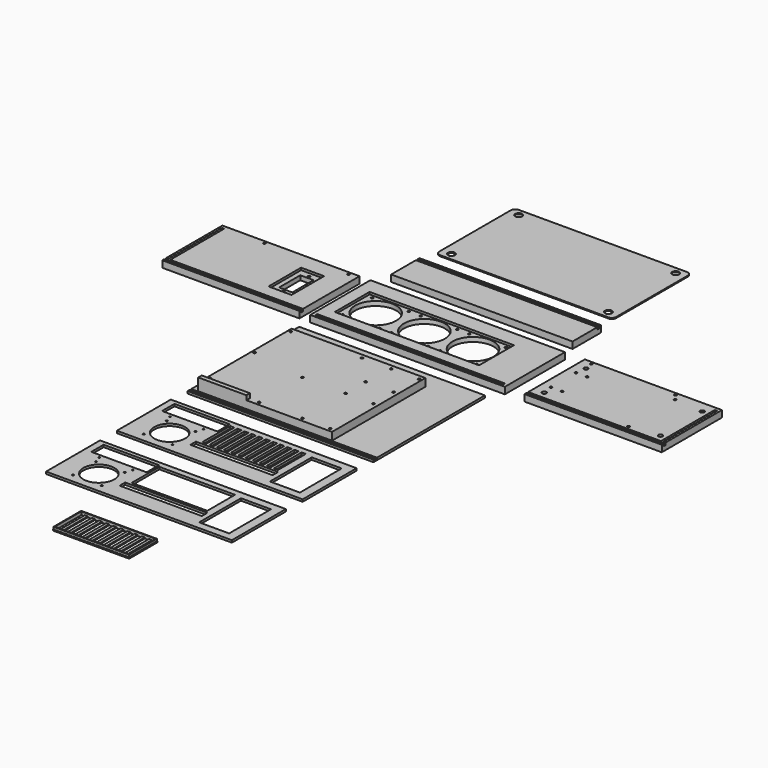
from build123d import *

# Parameters (mm, degrees)
F0_W      = 558.8
F0_H      = 215.9
F0_W_2    = 539.75
F0_H_2    = 6.5278
F0_W_3    = 414.33164
F0_H_3    = 125
F0_R      = 3.1877
F0_R_2    = 59
F1_DEPTH  = 12.7
F2_DEPTH  = 6.35
F3_R      = 6
F3_R_2    = 3.302
F3_W      = 393.7
F3_H      = 6.35
F3_W_2    = 6.3754
F3_H_2    = 2.8363937142
F3_H_3    = 193.4972
F4_DEPTH  = 12.7
F5_DEPTH  = 6.35
F6_R      = 3.302
F6_W      = 66.04
F6_H      = 116.84
F6_W_2    = 38.1
F6_H_2    = 76.2
F6_W_3    = 393.7
F6_H_3    = 6.35
F6_W_4    = 6.3754
F6_H_4    = 193.4972
F6_H_5    = 3.974708319
F7_DEPTH  = 12.7
F8_DEPTH  = 6.35
F9_DEPTH  = 6.35
F10_R     = 3.302
F10_W     = 138.0889187211
F10_H     = 12.6182494217
F11_DEPTH = 25.4
F12_DEPTH = 38.1
F13_W     = 533.4
F13_H     = 387.1722
F13_R     = 3.302
F13_H_2   = 6.5278
F13_H_3   = 6.35
F14_DEPTH = 3.2
F15_DEPTH = 3.2
F16_W     = 533.4
F16_H     = 193.6500064
F16_R     = 2.5
F16_R_2   = 44.5
F16_W_2   = 236.050014
F16_H_2   = 20
F16_R_3   = 2.0970704069
F16_R_4   = 2.1817303996
F16_W_3   = 12.0000014
F16_H_3   = 99.38
F16_W_4   = 158.75
F16_H_4   = 44.45
F16_W_5   = 12
F16_W_6   = 86
F16_H_5   = 150
F17_DEPTH = 6.3754
F18_W     = 520.7
F18_H     = 88.7222
F18_H_2   = 6.5278
F18_H_3   = 6.35
F19_DEPTH = 12.7
F20_DEPTH = 6.35
F21_R     = 10
F22_DEPTH = 3
F23_W     = 533.4
F23_H     = 193.6500064
F23_R     = 2.5
F23_R_2   = 44.5
F23_W_2   = 236.050014
F23_H_2   = 20
F23_R_3   = 2.0970704069
F23_R_4   = 2.1817303996
F23_W_3   = 158.75
F23_H_3   = 44.45
F23_W_4   = 217.000014
F23_H_4   = 99.38
F23_W_5   = 86
F23_H_5   = 150
F24_DEPTH = 6.3754
F25_W     = 219.000014
F25_H     = 101.3799892
F25_W_2   = 217.000014
F25_H_2   = 99.3799892
F25_W_3   = 8.5000084
F25_H_3   = 95.3799892
F25_W_4   = 8.499923
F26_DEPTH = 3
F27_DEPTH = 9.4


# Not quite as in the source:
# - a feature names something its author has since deleted; it is built from what else it names


with BuildPart() as f1:
    # F0 (on Top) → F1 (new body)
    with BuildSketch(Plane.XY):
        Rectangle(F0_W, F0_H)
        with Locations((0, -98.3361)):
            Rectangle(F0_W_2, F0_H_2, mode=Mode.SUBTRACT)
        with Locations((-38.1, 0)):
            Rectangle(F0_W_3, F0_H_3, mode=Mode.SUBTRACT)
        with Locations((-38.1, 0)):
            Rectangle(F0_W_3, F0_H_3)
        with Locations((-230.3, -52.5)):
            Circle(F0_R, mode=Mode.SUBTRACT)
        with Locations((-125.3, -52.5)):
            Circle(F0_R, mode=Mode.SUBTRACT)
        with Locations((-90.6, -52.5)):
            Circle(F0_R, mode=Mode.SUBTRACT)
        with Locations((14.4, -52.5)):
            Circle(F0_R, mode=Mode.SUBTRACT)
        with Locations((49.1, -52.5)):
            Circle(F0_R, mode=Mode.SUBTRACT)
        with Locations((154.1, -52.5)):
            Circle(F0_R, mode=Mode.SUBTRACT)
        with Locations((-177.8, 0)):
            Circle(F0_R_2, mode=Mode.SUBTRACT)
        with Locations((-230.3, 52.5)):
            Circle(F0_R, mode=Mode.SUBTRACT)
        with Locations((-38.1, 0)):
            Circle(F0_R_2, mode=Mode.SUBTRACT)
        with Locations((-125.3, 52.5)):
            Circle(F0_R, mode=Mode.SUBTRACT)
        with Locations((-90.6, 52.5)):
            Circle(F0_R, mode=Mode.SUBTRACT)
        with Locations((101.6, 0)):
            Circle(F0_R_2, mode=Mode.SUBTRACT)
        with Locations((14.4, 52.5)):
            Circle(F0_R, mode=Mode.SUBTRACT)
        with Locations((49.1, 52.5)):
            Circle(F0_R, mode=Mode.SUBTRACT)
        with Locations((154.1, 52.5)):
            Circle(F0_R, mode=Mode.SUBTRACT)
        with Locations((0, -98.3361)):
            Rectangle(F0_W_2, F0_H_2)
    extrude(amount=-F1_DEPTH)

    # F0 (on Top) → F2 (join)
    with BuildSketch(Plane.XY):
        Rectangle(F0_W, F0_H)
        with Locations((0, -98.3361)):
            Rectangle(F0_W_2, F0_H_2, mode=Mode.SUBTRACT)
        with Locations((-38.1, 0)):
            Rectangle(F0_W_3, F0_H_3, mode=Mode.SUBTRACT)
    extrude(amount=F2_DEPTH)


with BuildPart() as f4:
    # F3 (on Top) → F4 (new body)
    with BuildSketch(Plane.XY):
        Polygon((336.1011743546, 107.95), (336.1011743546, -95.0722), (717.0757743546, -95.0722), (717.0757743546, 98.425), (723.4511743546, 98.425), (723.4511743546, -95.0722), (729.8011743546, -95.0722), (729.8011743546, 107.95), align=None)
        with Locations((366.1011743546, -74.95)):
            Circle(F3_R, mode=Mode.SUBTRACT)
        with BuildLine():
            Line((389.9992377546, -45.0850025), (364.8031743546, -45.0850025))
            ThreePointArc((364.8031743546, -45.0850025), (359.1663077631, -47.4198690915), (361.5011743546, -41.7830025))
            Line((361.5011743546, -41.7830025), (361.5011743546, 41.7829975))
            ThreePointArc((361.5011743546, 41.7829975), (359.1663077631, 47.4198640915), (364.8031743546, 45.0849975))
            Line((364.8031743546, 45.0849975), (389.9992377546, 45.0849975))
            ThreePointArc((389.9992377546, 45.0849975), (393.3012377546, 48.3869975), (396.6032377546, 45.0849975))
            ThreePointArc((396.6032377546, 45.0849975), (395.636104346, 42.7501309085), (393.3012377546, 41.7829975))
            Line((393.3012377546, 41.7829975), (393.3012377546, -41.7830025))
            ThreePointArc((393.3012377546, -41.7830025), (395.636104346, -42.7501359085), (396.6032377546, -45.0850025))
            ThreePointArc((396.6032377546, -45.0850025), (393.3012377546, -48.3870025), (389.9992377546, -45.0850025))
        make_face(mode=Mode.SUBTRACT)
        with Locations((616.0757743546, -85.4085937142)):
            Circle(F3_R_2, mode=Mode.SUBTRACT)
        with Locations((699.8011743546, -74.95)):
            Circle(F3_R, mode=Mode.SUBTRACT)
        with Locations((366.1011743546, 74.95)):
            Circle(F3_R, mode=Mode.SUBTRACT)
        with Locations((361.5011743546, 99.95)):
            Circle(F3_R_2, mode=Mode.SUBTRACT)
        with Locations((616.0757743546, 81.95)):
            Circle(F3_R_2, mode=Mode.SUBTRACT)
        with Locations((602.8011743546, 99.95)):
            Circle(F3_R_2, mode=Mode.SUBTRACT)
        with Locations((699.8011743546, 74.95)):
            Circle(F3_R, mode=Mode.SUBTRACT)
        Polygon((336.1011743546, -95.0722), (336.1011743546, -101.6), (729.8011743546, -101.6), (729.8011743546, -95.0722), (723.4511743546, -95.0722), (723.4511743546, -97.9085937142), (717.0757743546, -97.9085937142), (717.0757743546, -95.0722), align=None)
        with Locations((532.9511743546, -104.775)):
            Rectangle(F3_W, F3_H)
        with Locations((720.2634743546, -96.4903968571)):
            Rectangle(F3_W_2, F3_H_2)
        with Locations((720.2634743546, 1.6764)):
            Rectangle(F3_W_2, F3_H_3)
        with Locations((366.1011743546, 74.95)):
            Circle(F3_R)
        with Locations((366.1011743546, 74.95)):
            Circle(F3_R_2, mode=Mode.SUBTRACT)
        with Locations((366.1011743546, -74.95)):
            Circle(F3_R)
        with Locations((366.1011743546, -74.95)):
            Circle(F3_R_2, mode=Mode.SUBTRACT)
        with Locations((699.8011743546, -74.95)):
            Circle(F3_R)
        with Locations((699.8011743546, -74.95)):
            Circle(F3_R_2, mode=Mode.SUBTRACT)
        with Locations((699.8011743546, 74.95)):
            Circle(F3_R)
        with Locations((699.8011743546, 74.95)):
            Circle(F3_R_2, mode=Mode.SUBTRACT)
        with BuildLine():
            ThreePointArc((361.5011743546, -41.7830025), (363.836040946, -42.7501359085), (364.8031743546, -45.0850025))
            Line((364.8031743546, -45.0850025), (389.9992377546, -45.0850025))
            ThreePointArc((389.9992377546, -45.0850025), (390.9663711631, -42.7501359085), (393.3012377546, -41.7830025))
            Line((393.3012377546, -41.7830025), (393.3012377546, 41.7829975))
            ThreePointArc((393.3012377546, 41.7829975), (390.9663711631, 42.7501309085), (389.9992377546, 45.0849975))
            Line((389.9992377546, 45.0849975), (364.8031743546, 45.0849975))
            ThreePointArc((364.8031743546, 45.0849975), (363.836040946, 42.7501309085), (361.5011743546, 41.7829975))
            Line((361.5011743546, 41.7829975), (361.5011743546, -41.7830025))
        make_face()
    extrude(amount=-F4_DEPTH)

    # F3 (on Top) → F5 (join)
    with BuildSketch(Plane.XY):
        Polygon((336.1011743546, 107.95), (336.1011743546, -95.0722), (717.0757743546, -95.0722), (717.0757743546, 98.425), (723.4511743546, 98.425), (723.4511743546, -95.0722), (729.8011743546, -95.0722), (729.8011743546, 107.95), align=None)
        with Locations((366.1011743546, -74.95)):
            Circle(F3_R, mode=Mode.SUBTRACT)
        with BuildLine():
            Line((389.9992377546, -45.0850025), (364.8031743546, -45.0850025))
            ThreePointArc((364.8031743546, -45.0850025), (359.1663077631, -47.4198690915), (361.5011743546, -41.7830025))
            Line((361.5011743546, -41.7830025), (361.5011743546, 41.7829975))
            ThreePointArc((361.5011743546, 41.7829975), (359.1663077631, 47.4198640915), (364.8031743546, 45.0849975))
            Line((364.8031743546, 45.0849975), (389.9992377546, 45.0849975))
            ThreePointArc((389.9992377546, 45.0849975), (393.3012377546, 48.3869975), (396.6032377546, 45.0849975))
            ThreePointArc((396.6032377546, 45.0849975), (395.636104346, 42.7501309085), (393.3012377546, 41.7829975))
            Line((393.3012377546, 41.7829975), (393.3012377546, -41.7830025))
            ThreePointArc((393.3012377546, -41.7830025), (395.636104346, -42.7501359085), (396.6032377546, -45.0850025))
            ThreePointArc((396.6032377546, -45.0850025), (393.3012377546, -48.3870025), (389.9992377546, -45.0850025))
        make_face(mode=Mode.SUBTRACT)
        with Locations((616.0757743546, -85.4085937142)):
            Circle(F3_R_2, mode=Mode.SUBTRACT)
        with Locations((699.8011743546, -74.95)):
            Circle(F3_R, mode=Mode.SUBTRACT)
        with Locations((366.1011743546, 74.95)):
            Circle(F3_R, mode=Mode.SUBTRACT)
        with Locations((361.5011743546, 99.95)):
            Circle(F3_R_2, mode=Mode.SUBTRACT)
        with Locations((616.0757743546, 81.95)):
            Circle(F3_R_2, mode=Mode.SUBTRACT)
        with Locations((602.8011743546, 99.95)):
            Circle(F3_R_2, mode=Mode.SUBTRACT)
        with Locations((699.8011743546, 74.95)):
            Circle(F3_R, mode=Mode.SUBTRACT)
        with Locations((532.9511743546, -104.775)):
            Rectangle(F3_W, F3_H)
        with BuildLine():
            ThreePointArc((361.5011743546, -41.7830025), (363.836040946, -42.7501359085), (364.8031743546, -45.0850025))
            Line((364.8031743546, -45.0850025), (389.9992377546, -45.0850025))
            ThreePointArc((389.9992377546, -45.0850025), (390.9663711631, -42.7501359085), (393.3012377546, -41.7830025))
            Line((393.3012377546, -41.7830025), (393.3012377546, 41.7829975))
            ThreePointArc((393.3012377546, 41.7829975), (390.9663711631, 42.7501309085), (389.9992377546, 45.0849975))
            Line((389.9992377546, 45.0849975), (364.8031743546, 45.0849975))
            ThreePointArc((364.8031743546, 45.0849975), (363.836040946, 42.7501309085), (361.5011743546, 41.7829975))
            Line((361.5011743546, 41.7829975), (361.5011743546, -41.7830025))
        make_face()
    extrude(amount=F5_DEPTH)


with BuildPart() as f7:
    # F6 (on Top) → F7 (new body)
    with BuildSketch(Plane.XY):
        Polygon((-310.4593753815, -95.0722), (-310.4593753815, 107.95), (-704.1593753815, 107.95), (-704.1593753815, -95.0722), (-697.8093753815, -95.0722), (-697.8093753815, 98.425), (-691.4339753815, 98.425), (-691.4339753815, -95.0722), align=None)
        with Locations((-577.1593753815, 99.95)):
            Circle(F6_R, mode=Mode.SUBTRACT)
        with Locations((-405.7093753815, 0)):
            Rectangle(F6_W, F6_H, mode=Mode.SUBTRACT)
        with Locations((-335.8593753815, 99.95)):
            Circle(F6_R, mode=Mode.SUBTRACT)
        with Locations((-405.7093753815, 0)):
            Rectangle(F6_W, F6_H)
        with Locations((-405.7093753815, -45.6)):
            Circle(F6_R, mode=Mode.SUBTRACT)
        with Locations((-405.7093753815, 0)):
            Rectangle(F6_W_2, F6_H_2, mode=Mode.SUBTRACT)
        with Locations((-405.7093753815, 45.6)):
            Circle(F6_R, mode=Mode.SUBTRACT)
        Polygon((-310.4593753815, -101.6), (-310.4593753815, -95.0722), (-691.4339753815, -95.0722), (-691.4339753815, -99.046908319), (-697.8093753815, -99.046908319), (-697.8093753815, -95.0722), (-704.1593753815, -95.0722), (-704.1593753815, -101.6), align=None)
        with Locations((-507.3093753815, -104.775)):
            Rectangle(F6_W_3, F6_H_3)
        with Locations((-694.6216753815, 1.6764)):
            Rectangle(F6_W_4, F6_H_4)
        with Locations((-694.6216753815, -97.0595541595)):
            Rectangle(F6_W_4, F6_H_5)
    extrude(amount=-F7_DEPTH)

    # F6 (on Top) → F8 (join)
    with BuildSketch(Plane.XY):
        Polygon((-310.4593753815, -95.0722), (-310.4593753815, 107.95), (-704.1593753815, 107.95), (-704.1593753815, -95.0722), (-697.8093753815, -95.0722), (-697.8093753815, 98.425), (-691.4339753815, 98.425), (-691.4339753815, -95.0722), align=None)
        with Locations((-577.1593753815, 99.95)):
            Circle(F6_R, mode=Mode.SUBTRACT)
        with Locations((-405.7093753815, 0)):
            Rectangle(F6_W, F6_H, mode=Mode.SUBTRACT)
        with Locations((-335.8593753815, 99.95)):
            Circle(F6_R, mode=Mode.SUBTRACT)
        with Locations((-405.7093753815, 0)):
            Rectangle(F6_W, F6_H)
        with Locations((-405.7093753815, -45.6)):
            Circle(F6_R, mode=Mode.SUBTRACT)
        with Locations((-405.7093753815, 0)):
            Rectangle(F6_W_2, F6_H_2, mode=Mode.SUBTRACT)
        with Locations((-405.7093753815, 45.6)):
            Circle(F6_R, mode=Mode.SUBTRACT)
        with Locations((-507.3093753815, -104.775)):
            Rectangle(F6_W_3, F6_H_3)
    extrude(amount=F8_DEPTH)

    # F6 (on Top) → F9 (cut)
    with BuildSketch(Plane.XY):
        with Locations((-405.7093753815, 0)):
            Rectangle(F6_W, F6_H)
        with Locations((-405.7093753815, -45.6)):
            Circle(F6_R, mode=Mode.SUBTRACT)
        with Locations((-405.7093753815, 0)):
            Rectangle(F6_W_2, F6_H_2, mode=Mode.SUBTRACT)
        with Locations((-405.7093753815, 45.6)):
            Circle(F6_R, mode=Mode.SUBTRACT)
    extrude(amount=F9_DEPTH, mode=Mode.SUBTRACT)


with BuildPart() as f11:
    # F10 (on Top) → F11 (new body)
    with BuildSketch(Plane.XY):
        Polygon((136.35, -549.4468963333), (136.35, -214.4468963333), (-247.65, -214.4468963333), (-247.65, -536.8286469116), (-109.5610812789, -536.8286469116), (-109.5610812789, -549.4468963333), align=None)
        with Locations((-239.65, -517.4468963333)):
            Circle(F10_R, mode=Mode.SUBTRACT)
        with Locations((-80.65, -539.4468963333)):
            Circle(F10_R, mode=Mode.SUBTRACT)
        with Locations((-80.65, -384.4468963333)):
            Circle(F10_R, mode=Mode.SUBTRACT)
        with Locations((43.35, -539.4468963333)):
            Circle(F10_R, mode=Mode.SUBTRACT)
        with Locations((123.35, -539.4468963333)):
            Circle(F10_R, mode=Mode.SUBTRACT)
        with Locations((43.3500082, -384.4468963333)):
            Circle(F10_R, mode=Mode.SUBTRACT)
        with Locations((123.35, -384.4468963333)):
            Circle(F10_R, mode=Mode.SUBTRACT)
        with Locations((-239.65, -357.4468963333)):
            Circle(F10_R, mode=Mode.SUBTRACT)
        with Locations((-239.65, -227.4468963333)):
            Circle(F10_R, mode=Mode.SUBTRACT)
        with Locations((43.3500082, -312.4468963333)):
            Circle(F10_R, mode=Mode.SUBTRACT)
        with Locations((123.35, -312.4468963333)):
            Circle(F10_R, mode=Mode.SUBTRACT)
        with Locations((-35.15, -227.4468963333)):
            Circle(F10_R, mode=Mode.SUBTRACT)
        with Locations((48.85, -227.4468963333)):
            Circle(F10_R, mode=Mode.SUBTRACT)
        with Locations((128.85, -227.4468963333)):
            Circle(F10_R, mode=Mode.SUBTRACT)
        with Locations((-178.6055406395, -543.1377716225)):
            Rectangle(F10_W, F10_H)
    extrude(amount=F11_DEPTH)

    # F10 (on Top) → F12 (join)
    with BuildSketch(Plane.XY):
        with Locations((-178.6055406395, -543.1377716225)):
            Rectangle(F10_W, F10_H)
    extrude(amount=F12_DEPTH)


with BuildPart() as f14:
    # F13 (on Top) → F14 (new body)
    with BuildSketch(Plane.XY):
        with Locations((0, -357.2083963333)):
            Rectangle(F13_W, F13_H)
        with Locations((-239.65, -517.4468963333)):
            Circle(F13_R, mode=Mode.SUBTRACT)
        with Locations((-80.65, -539.4468963333)):
            Circle(F13_R, mode=Mode.SUBTRACT)
        with Locations((-80.65, -384.4468963333)):
            Circle(F13_R, mode=Mode.SUBTRACT)
        with Locations((43.35, -539.4468963333)):
            Circle(F13_R, mode=Mode.SUBTRACT)
        with Locations((123.35, -539.4468963333)):
            Circle(F13_R, mode=Mode.SUBTRACT)
        with Locations((43.3500082, -384.4468963333)):
            Circle(F13_R, mode=Mode.SUBTRACT)
        with Locations((123.35, -384.4468963333)):
            Circle(F13_R, mode=Mode.SUBTRACT)
        with Locations((-239.65, -357.4468963333)):
            Circle(F13_R, mode=Mode.SUBTRACT)
        with Locations((-239.65, -227.4468963333)):
            Circle(F13_R, mode=Mode.SUBTRACT)
        with Locations((-35.15, -227.4468963333)):
            Circle(F13_R, mode=Mode.SUBTRACT)
        with Locations((43.3500082, -312.4468963333)):
            Circle(F13_R, mode=Mode.SUBTRACT)
        with Locations((123.35, -312.4468963333)):
            Circle(F13_R, mode=Mode.SUBTRACT)
        with Locations((48.85, -227.4468963333)):
            Circle(F13_R, mode=Mode.SUBTRACT)
        with Locations((128.85, -227.4468963333)):
            Circle(F13_R, mode=Mode.SUBTRACT)
        with Locations((0, -554.0583963333)):
            Rectangle(F13_W, F13_H_2)
        with Locations((0, -560.4972963333)):
            Rectangle(F13_W, F13_H_3)
    extrude(amount=-F14_DEPTH)

    # F13 (on Top) → F15 (join)
    with BuildSketch(Plane.XY):
        with Locations((0, -357.2083963333)):
            Rectangle(F13_W, F13_H)
        with Locations((-239.65, -517.4468963333)):
            Circle(F13_R, mode=Mode.SUBTRACT)
        with Locations((-80.65, -539.4468963333)):
            Circle(F13_R, mode=Mode.SUBTRACT)
        with Locations((-80.65, -384.4468963333)):
            Circle(F13_R, mode=Mode.SUBTRACT)
        with Locations((43.35, -539.4468963333)):
            Circle(F13_R, mode=Mode.SUBTRACT)
        with Locations((123.35, -539.4468963333)):
            Circle(F13_R, mode=Mode.SUBTRACT)
        with Locations((43.3500082, -384.4468963333)):
            Circle(F13_R, mode=Mode.SUBTRACT)
        with Locations((123.35, -384.4468963333)):
            Circle(F13_R, mode=Mode.SUBTRACT)
        with Locations((-239.65, -357.4468963333)):
            Circle(F13_R, mode=Mode.SUBTRACT)
        with Locations((-239.65, -227.4468963333)):
            Circle(F13_R, mode=Mode.SUBTRACT)
        with Locations((-35.15, -227.4468963333)):
            Circle(F13_R, mode=Mode.SUBTRACT)
        with Locations((43.3500082, -312.4468963333)):
            Circle(F13_R, mode=Mode.SUBTRACT)
        with Locations((123.35, -312.4468963333)):
            Circle(F13_R, mode=Mode.SUBTRACT)
        with Locations((48.85, -227.4468963333)):
            Circle(F13_R, mode=Mode.SUBTRACT)
        with Locations((128.85, -227.4468963333)):
            Circle(F13_R, mode=Mode.SUBTRACT)
        with Locations((0, -560.4972963333)):
            Rectangle(F13_W, F13_H_3)
    extrude(amount=F15_DEPTH)


with BuildPart() as f17:
    # F16 (on Top) → F17 (new body)
    with BuildSketch(Plane.XY):
        with Locations((0, -720.8472931333)):
            Rectangle(F16_W, F16_H)
        with Locations((-209.1694, -792.8822963333)):
            Circle(F16_R, mode=Mode.SUBTRACT)
        with Locations((-126.6694, -792.8822963333)):
            Circle(F16_R, mode=Mode.SUBTRACT)
        with Locations((-167.9194, -751.6322963333)):
            Circle(F16_R_2, mode=Mode.SUBTRACT)
        with Locations((22.77498286, -758.2222783933)):
            Rectangle(F16_W_2, F16_H_2, mode=Mode.SUBTRACT)
        with Locations((-209.1694, -710.3822963333)):
            Circle(F16_R, mode=Mode.SUBTRACT)
        with Locations((-216.02501754, -690.1722947933)):
            Circle(F16_R_3, mode=Mode.SUBTRACT)
        with Locations((-126.6694, -710.3822963333)):
            Circle(F16_R, mode=Mode.SUBTRACT)
        with Locations((-119.82500674, -690.1722947933)):
            Circle(F16_R_4, mode=Mode.SUBTRACT)
        with Locations((-76.55002344, -690.9122783933)):
            Rectangle(F16_W_3, F16_H_3, mode=Mode.SUBTRACT)
        with Locations((-56.05002204, -690.9122783933)):
            Rectangle(F16_W_3, F16_H_3, mode=Mode.SUBTRACT)
        with Locations((-35.55002064, -690.9122783933)):
            Rectangle(F16_W_3, F16_H_3, mode=Mode.SUBTRACT)
        with Locations((-15.05001924, -690.9122783933)):
            Rectangle(F16_W_3, F16_H_3, mode=Mode.SUBTRACT)
        with Locations((-167.92501214, -657.4472903933)):
            Rectangle(F16_W_4, F16_H_4, mode=Mode.SUBTRACT)
        with Locations((5.44998216, -690.9122783933)):
            Rectangle(F16_W_3, F16_H_3, mode=Mode.SUBTRACT)
        with Locations((25.94998356, -690.9122783933)):
            Rectangle(F16_W_3, F16_H_3, mode=Mode.SUBTRACT)
        with Locations((46.44998496, -690.9122783933)):
            Rectangle(F16_W_3, F16_H_3, mode=Mode.SUBTRACT)
        with Locations((66.94998636, -690.9122783933)):
            Rectangle(F16_W_3, F16_H_3, mode=Mode.SUBTRACT)
        with Locations((87.44998776, -690.9122783933)):
            Rectangle(F16_W_3, F16_H_3, mode=Mode.SUBTRACT)
        with Locations((107.94998916, -690.9122783933)):
            Rectangle(F16_W_3, F16_H_3, mode=Mode.SUBTRACT)
        with Locations((128.44998986, -690.9122783933)):
            Rectangle(F16_W_5, F16_H_3, mode=Mode.SUBTRACT)
        with Locations((198.3, -720.8472931333)):
            Rectangle(F16_W_6, F16_H_5, mode=Mode.SUBTRACT)
    extrude(amount=F17_DEPTH)


with BuildPart() as f19:
    # F18 (on Top) → F19 (new body)
    with BuildSketch(Plane.XY):
        with Locations((0, 203.1111)):
            Rectangle(F18_W, F18_H)
        with Locations((0, 250.7361)):
            Rectangle(F18_W, F18_H_2)
        with Locations((0, 257.175)):
            Rectangle(F18_W, F18_H_3)
    extrude(amount=-F19_DEPTH)

    # F18 (on Top) → F20 (join)
    with BuildSketch(Plane.XY):
        with Locations((0, 257.175)):
            Rectangle(F18_W, F18_H_3)
        with Locations((0, 203.1111)):
            Rectangle(F18_W, F18_H)
    extrude(amount=F20_DEPTH)


with BuildPart() as f22:
    # F21 (on Top) → F22 (new body)
    with BuildSketch(Plane.XY):
        with BuildLine():
            ThreePointArc((-249.73, 318.2267664064), (-246.0102561211, 309.2465102853), (-237.03, 305.5267664064))
            Line((-237.03, 305.5267664064), (245.57, 305.5267664064))
            ThreePointArc((245.57, 305.5267664064), (254.5502561211, 309.2465102853), (258.27, 318.2267664064))
            Line((258.27, 318.2267664064), (258.27, 574.7667664064))
            ThreePointArc((258.27, 574.7667664064), (254.5502561211, 583.7470225275), (245.57, 587.4667664064))
            Line((245.57, 587.4667664064), (-237.03, 587.4667664064))
            ThreePointArc((-237.03, 587.4667664064), (-246.0102561211, 583.7470225275), (-249.73, 574.7667664064))
            Line((-249.73, 574.7667664064), (-249.73, 318.2267664064))
        make_face()
        with Locations((-221.0799938, 325.8467664064)):
            Circle(F21_R, mode=Mode.SUBTRACT)
        with Locations((229.6200062, 325.8467664064)):
            Circle(F21_R, mode=Mode.SUBTRACT)
        with Locations((-221.0799938, 567.1467664064)):
            Circle(F21_R, mode=Mode.SUBTRACT)
        with Locations((229.6200062, 567.1467664064)):
            Circle(F21_R, mode=Mode.SUBTRACT)
    extrude(amount=F22_DEPTH)


with BuildPart() as f24:
    # F23 (on Top) → F24 (new body)
    with BuildSketch(Plane.XY):
        with Locations((0, -974.8472931333)):
            Rectangle(F23_W, F23_H)
        with Locations((-209.1694, -1046.8822963333)):
            Circle(F23_R, mode=Mode.SUBTRACT)
        with Locations((-126.6694, -1046.8822963333)):
            Circle(F23_R, mode=Mode.SUBTRACT)
        with Locations((-167.9194, -1005.6322963333)):
            Circle(F23_R_2, mode=Mode.SUBTRACT)
        with Locations((22.77498286, -1012.2222783933)):
            Rectangle(F23_W_2, F23_H_2, mode=Mode.SUBTRACT)
        with Locations((-209.1694, -964.3822963333)):
            Circle(F23_R, mode=Mode.SUBTRACT)
        with Locations((-216.02501754, -944.1722947933)):
            Circle(F23_R_3, mode=Mode.SUBTRACT)
        with Locations((-126.6694, -964.3822963333)):
            Circle(F23_R, mode=Mode.SUBTRACT)
        with Locations((-119.82500674, -944.1722947933)):
            Circle(F23_R_4, mode=Mode.SUBTRACT)
        with Locations((-167.92501214, -911.4472903933)):
            Rectangle(F23_W_3, F23_H_3, mode=Mode.SUBTRACT)
        with Locations((25.94998286, -944.9122783933)):
            Rectangle(F23_W_4, F23_H_4, mode=Mode.SUBTRACT)
        with Locations((198.3, -974.8472931333)):
            Rectangle(F23_W_5, F23_H_5, mode=Mode.SUBTRACT)
    extrude(amount=F24_DEPTH)


with BuildPart() as f26:
    # F25 (on Top) → F26 (new body)
    with BuildSketch(Plane.XY):
        with Locations((25.94998286, -1225.6019718383)):
            Rectangle(F25_W, F25_H)
        with Locations((25.94998286, -1225.6019718383)):
            Rectangle(F25_W_2, F25_H_2, mode=Mode.SUBTRACT)
        with Locations((25.94998286, -1225.6019718383)):
            Rectangle(F25_W_2, F25_H_2)
        Polygon((-80.55002414, -1273.2919664383), (-80.55002414, -1177.9119772383), (-70.55002274, -1177.9119772383), (-62.05001434, -1177.9119772383), (-50.05001294, -1177.9119772383), (-41.55000454, -1177.9119772383), (-29.55000314, -1177.9119772383), (-21.04999474, -1177.9119772383), (-9.04999334, -1177.9119772383), (-0.54998494, -1177.9119772383), (11.45001646, -1177.9119772383), (19.95002486, -1177.9119772383), (31.95002626, -1177.9119772383), (40.45003466, -1177.9119772383), (52.45003606, -1177.9119772383), (60.95004446, -1177.9119772383), (72.95004586, -1177.9119772383), (81.45005426, -1177.9119772383), (93.45005566, -1177.9119772383), (101.94997866, -1177.9119772383), (113.94998006, -1177.9119772383), (122.44998846, -1177.9119772383), (132.44998986, -1177.9119772383), (132.44998986, -1273.2919664383), (122.44998846, -1273.2919664383), (113.94998006, -1273.2919664383), (101.94997866, -1273.2919664383), (93.45005566, -1273.2919664383), (81.45005426, -1273.2919664383), (72.95004586, -1273.2919664383), (60.95004446, -1273.2919664383), (52.45003606, -1273.2919664383), (40.45003466, -1273.2919664383), (31.95002626, -1273.2919664383), (19.95002486, -1273.2919664383), (11.45001646, -1273.2919664383), (-0.54998494, -1273.2919664383), (-9.04999334, -1273.2919664383), (-21.04999474, -1273.2919664383), (-29.55000314, -1273.2919664383), (-41.55000454, -1273.2919664383), (-50.05001294, -1273.2919664383), (-62.05001434, -1273.2919664383), (-70.55002274, -1273.2919664383), align=None, mode=Mode.SUBTRACT)
        with Locations((-66.30001854, -1225.6019718383)):
            Rectangle(F25_W_3, F25_H_3)
        with Locations((-45.80000874, -1225.6019718383)):
            Rectangle(F25_W_3, F25_H_3)
        with Locations((-25.29999894, -1225.6019718383)):
            Rectangle(F25_W_3, F25_H_3)
        with Locations((-4.79998914, -1225.6019718383)):
            Rectangle(F25_W_3, F25_H_3)
        with Locations((15.70002066, -1225.6019718383)):
            Rectangle(F25_W_3, F25_H_3)
        with Locations((36.20003046, -1225.6019718383)):
            Rectangle(F25_W_3, F25_H_3)
        with Locations((56.70004026, -1225.6019718383)):
            Rectangle(F25_W_3, F25_H_3)
        with Locations((77.20005006, -1225.6019718383)):
            Rectangle(F25_W_3, F25_H_3)
        with Locations((118.19998426, -1225.6019718383)):
            Rectangle(F25_W_3, F25_H_3)
        with Locations((97.70001716, -1225.6019718383)):
            Rectangle(F25_W_4, F25_H_3)
    extrude(amount=F26_DEPTH)

    # F25 (on Top) → F27 (join)
    with BuildSketch(Plane.XY):
        with Locations((25.94998286, -1225.6019718383)):
            Rectangle(F25_W_2, F25_H_2)
        Polygon((-80.55002414, -1273.2919664383), (-80.55002414, -1177.9119772383), (-70.55002274, -1177.9119772383), (-62.05001434, -1177.9119772383), (-50.05001294, -1177.9119772383), (-41.55000454, -1177.9119772383), (-29.55000314, -1177.9119772383), (-21.04999474, -1177.9119772383), (-9.04999334, -1177.9119772383), (-0.54998494, -1177.9119772383), (11.45001646, -1177.9119772383), (19.95002486, -1177.9119772383), (31.95002626, -1177.9119772383), (40.45003466, -1177.9119772383), (52.45003606, -1177.9119772383), (60.95004446, -1177.9119772383), (72.95004586, -1177.9119772383), (81.45005426, -1177.9119772383), (93.45005566, -1177.9119772383), (101.94997866, -1177.9119772383), (113.94998006, -1177.9119772383), (122.44998846, -1177.9119772383), (132.44998986, -1177.9119772383), (132.44998986, -1273.2919664383), (122.44998846, -1273.2919664383), (113.94998006, -1273.2919664383), (101.94997866, -1273.2919664383), (93.45005566, -1273.2919664383), (81.45005426, -1273.2919664383), (72.95004586, -1273.2919664383), (60.95004446, -1273.2919664383), (52.45003606, -1273.2919664383), (40.45003466, -1273.2919664383), (31.95002626, -1273.2919664383), (19.95002486, -1273.2919664383), (11.45001646, -1273.2919664383), (-0.54998494, -1273.2919664383), (-9.04999334, -1273.2919664383), (-21.04999474, -1273.2919664383), (-29.55000314, -1273.2919664383), (-41.55000454, -1273.2919664383), (-50.05001294, -1273.2919664383), (-62.05001434, -1273.2919664383), (-70.55002274, -1273.2919664383), align=None, mode=Mode.SUBTRACT)
    extrude(amount=F27_DEPTH)


solid = Compound([f1.part, f4.part, f7.part, f11.part, f14.part, f17.part, f19.part, f22.part, f24.part, f26.part])
